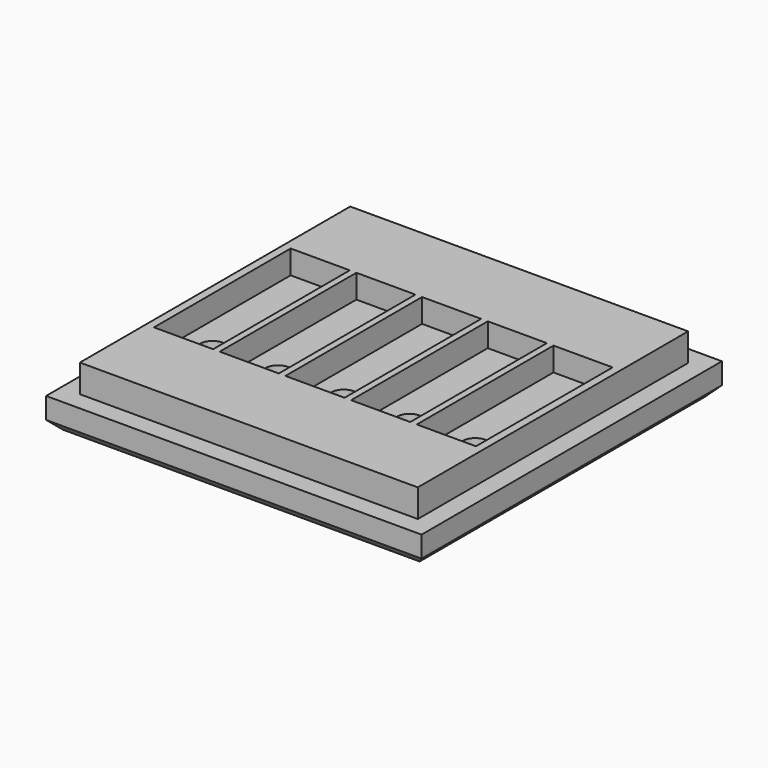
from build123d import *

# Parameters (mm, degrees)
F0_W      = 50.8
F0_H      = 50.8
F1_DEPTH  = 4.13
F3_W      = 45.72
F3_H      = 45.72
F4_DEPTH  = 3.77
F5_W      = 8
F5_H      = 23.114
F6_DEPTH  = 3.2
F7_R      = 1.715
F8_DEPTH  = 25.4
F9_SIZE   = 1.27
F10_R     = 1.694213851
F11_DEPTH = 25.4


# Not quite as in the source:
# - a feature names something its author has since deleted; it is built from what else it names


with BuildPart() as f1:
    # F0 (on Top) → F1 (new body)
    with BuildSketch(Plane.XY):
        with Locations((13.0843408406, 14.7212249442)):
            Rectangle(F0_W, F0_H)
    extrude(amount=F1_DEPTH)

    # F3 (on face) → F4 (join)
    with BuildSketch(Plane.XY.offset(4.13)):
        with Locations((13.0843408406, 14.7212249442)):
            Rectangle(F3_W, F3_H)
    extrude(amount=F4_DEPTH)

    # F5 (on face) → F6 (cut)
    with BuildSketch(Plane.XY.offset(7.9)):
        with Locations((4.2001288666, 14.5942249442)):
            Rectangle(F5_W, F5_H)
        with Locations((13.0901288666, 14.5942249442)):
            Rectangle(F5_W, F5_H)
        with Locations((21.9801288666, 14.5942249442)):
            Rectangle(F5_W, F5_H)
        with Locations((30.8701288666, 14.5942249442)):
            Rectangle(F5_W, F5_H)
        with Locations((-4.6898711334, 14.5942249442)):
            Rectangle(F5_W, F5_H)
    extrude(amount=-F6_DEPTH, mode=Mode.SUBTRACT)

    # F7 (on face) → F8 (cut)
    with BuildSketch(Plane.XY.offset(4.7)):
        with Locations((-4.6898711334, 7.9362249442)):
            Circle(F7_R)
    extrude(amount=-F8_DEPTH, mode=Mode.SUBTRACT)

    # F9
    f9_edges = [f1.edges().sort_by_distance(p)[0] for p in [
        (13.084341, -10.678775, 0),
        (13.084341, 40.121225, 0),
        (-12.315659, 14.721225, 0),
        (38.484341, 14.721225, 0),
    ]]
    chamfer(f9_edges, length=F9_SIZE)

    # F10 (on face) → F11 (cut)
    with BuildSketch(Plane.XY.offset(4.7)):
        with Locations((4.1879288666, 7.9312249442)):
            Circle(F10_R)
        with Locations((13.0779288666, 7.9312249442)):
            Circle(F10_R)
        with Locations((21.9679288666, 7.9312249442)):
            Circle(F10_R)
        with Locations((30.8579288666, 7.9394249442)):
            Circle(F10_R)
    extrude(amount=-F11_DEPTH, mode=Mode.SUBTRACT)


solid = f1.part
